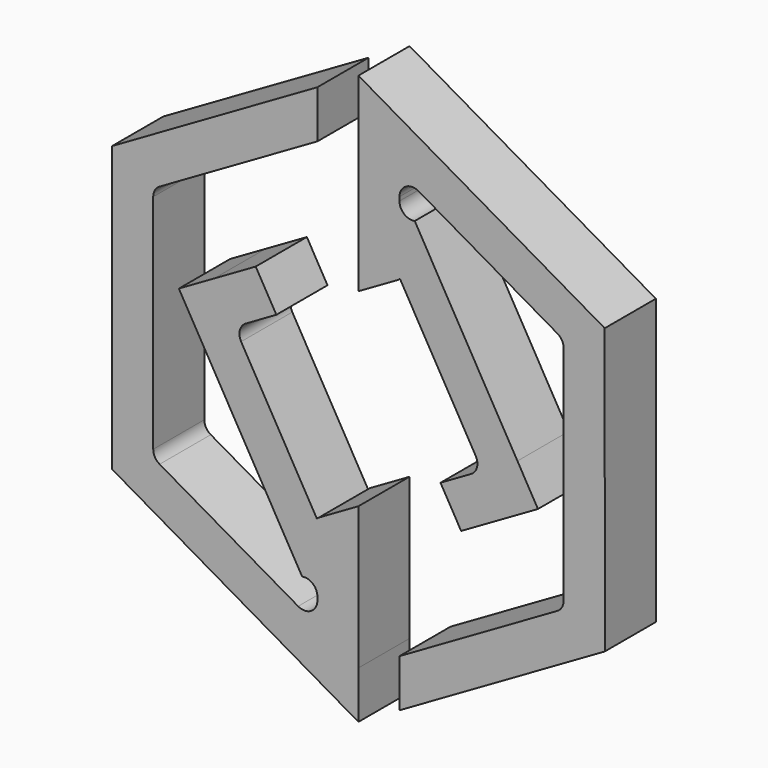
from build123d import *

# Parameters (mm, degrees)
F1_DEPTH      = 25.4
F2_T1_DEPTH   = 25.4
F2_T3_DEPTH   = 31.626178471
F2_2_T1_DEPTH = 25.4
F2_2_T3_DEPTH = 31.595918111


# Not quite as in the source:
# - a fillet or chamfer that OpenCascade refuses, or shapes differently, is made with other operations: its cross-section is extruded or revolved along the edge and cut away or added


with BuildPart() as f1:
    # F0 (on Front) → F1 (new body)
    with BuildSketch(Plane.XZ):
        Polygon((-16.319119, 103.6338542), (-97.871661, 56.5480962), (-97.834323, -56.4841898), (0.000889, -113.0128042), (-0.021209, -94.1582318), (-0.041783, -37.6147838), (-16.454247, -47.0889838), (-16.483203, -47.3297758), (-16.538321, -47.2350338), (-49.133125, 9.2218002), (-32.599503, 18.7691522), (-40.798877, 32.9710542), (-57.263665, 23.4681522), (-71.323581, 15.3475182), (-63.162815, 1.2154662), (-22.370161, -69.4435238), (-16.319119, -65.9487378), (-16.319119, -84.7493098), (-81.509997, -47.1080338), (-81.517109, 47.0517982), (-16.276447, 84.7189822), align=None)
    extrude(amount=F1_DEPTH)

    # F2: fillet of radius 5.08 on 6 edges, made by hand

    # F2_s2 → F2_t1 (join)
    with BuildSketch(Plane.XZ):
        with BuildLine():
            ThreePointArc((-78.9703857887, -48.5744077693), (-80.8295799283, -46.715177806), (-81.5102184992, -44.1754789968))
            Line((-81.5102184992, -44.1754789968), (-81.509997, -47.1080338))
            Line((-81.509997, -47.1080338), (-78.9703857887, -48.5744077693))
        make_face()
        with BuildLine():
            ThreePointArc((-16.319119, -75.9501053756), (-18.8592026389, -80.3495627147), (-23.939286275, -80.3494178464))
            Line((-23.939286275, -80.3494178464), (-16.319119, -84.7493098))
            Line((-16.319119, -84.7493098), (-16.319119, -75.9501053756))
        make_face()
        with BuildLine():
            ThreePointArc((-22.370161, -69.4435238), (-18.1685225659, -70.5094387585), (-16.319119, -74.4298528539))
            Line((-16.319119, -74.4298528539), (-16.319119, -65.9487378))
            Line((-16.319119, -65.9487378), (-22.370161, -69.4435238))
        make_face()
        with BuildLine():
            ThreePointArc((-81.5168874538, 44.1186213446), (-80.8363993057, 46.6588270036), (-78.9769112502, 48.5184003635))
            Line((-78.9769112502, 48.5184003635), (-81.517109, 47.0517982))
            Line((-81.517109, 47.0517982), (-81.5168874538, 44.1186213446))
        make_face()
        with BuildLine():
            ThreePointArc((-46.5933683691, 4.8227365177), (-47.1008880705, 8.6773378396), (-44.7342717126, 11.7619212171))
            Line((-44.7342717126, 11.7619212171), (-49.133125, 9.2218002))
            Line((-49.133125, 9.2218002), (-46.5933683691, 4.8227365177))
        make_face()
    extrude(amount=F2_T1_DEPTH)

    # F2_s4 → F2_t3 (cut)
    with BuildSketch(Plane.XZ.offset(-3.1130892355)):
        with BuildLine():
            ThreePointArc((-15.3757974258, -46.4664418736), (-15.9594734444, -46.8596619247), (-16.483203, -47.3297758))
            Line((-16.483203, -47.3297758), (-16.454247, -47.0889838))
            Line((-16.454247, -47.0889838), (-15.3757974258, -46.4664418736))
        make_face()
    extrude(amount=F2_T3_DEPTH, mode=Mode.SUBTRACT)


with BuildPart() as f1b:
    # F0 (on Front) → F1, piece 2 (new body)
    with BuildSketch(Plane.XZ):
        Polygon((16.316833, -103.6324318), (97.871661, -56.5476898), (97.836101, 56.4845962), (0.000889, 113.0128042), (0.021463, 94.1586382), (0.040767, 37.6151902), (16.451707, 47.0888822), (16.483457, 47.3301822), (16.537305, 47.2326462), (49.133379, -9.2246958), (32.599757, -18.7700158), (40.799131, -32.9709018), (57.261125, -23.4664758), (71.323835, -15.3499058), (63.164339, -1.2178538), (22.370669, 69.4408822), (16.316833, 65.9488902), (16.316833, 84.7479382), (81.507711, 47.1056462), (81.518633, -47.0516458), (16.278225, -84.7203538), align=None)
    extrude(amount=F1_DEPTH)

    # F2#2: fillet of radius 5.08 on 6 edges, made by hand

    # F2_2_s2 → F2_2_t1 (join)
    with BuildSketch(Plane.XZ):
        with BuildLine():
            ThreePointArc((46.5932982219, -4.8252024991), (47.1007988179, -8.6800552118), (44.7338290233, -11.7646784114))
            Line((44.7338290233, -11.7646784114), (49.133379, -9.2246958))
            Line((49.133379, -9.2246958), (46.5932982219, -4.8252024991))
        make_face()
        with BuildLine():
            ThreePointArc((16.316833, 75.9486150149), (18.8569423497, 80.3480871974), (23.9370516947, 80.3478977955))
            Line((23.9370516947, 80.3478977955), (16.316833, 84.7479382))
            Line((16.316833, 84.7479382), (16.316833, 75.9486150149))
        make_face()
        with BuildLine():
            ThreePointArc((22.370669, 69.4408822), (18.1673351195, 70.505347241), (16.316833, 74.4266663354))
            Line((16.316833, 74.4266663354), (16.316833, 65.9488902))
            Line((16.316833, 65.9488902), (22.370669, 69.4408822))
        make_face()
        with BuildLine():
            ThreePointArc((78.968269877, 48.5719615374), (80.8273760471, 46.7128245665), (81.5080511482, 44.1732680235))
            Line((81.5080511482, 44.1732680235), (81.507711, 47.1056462))
            Line((81.507711, 47.1056462), (78.968269877, 48.5719615374))
        make_face()
        with BuildLine():
            ThreePointArc((78.9784010584, -48.5183327536), (80.8378803981, -46.6586769125), (81.5182927508, -44.1183969491))
            Line((81.5182927508, -44.1183969491), (81.518633, -47.0516458))
            Line((81.518633, -47.0516458), (78.9784010584, -48.5183327536))
        make_face()
    extrude(amount=F2_2_T1_DEPTH)

    # F2_2_s4 → F2_2_t3 (cut)
    with BuildSketch(Plane.XZ.offset(-3.0979590555)):
        with BuildLine():
            ThreePointArc((15.3785094128, 46.4693477068), (15.9607949827, 46.861499235), (16.483457, 47.3301822))
            Line((16.483457, 47.3301822), (16.451707, 47.0888822))
            Line((16.451707, 47.0888822), (15.3785094128, 46.4693477068))
        make_face()
    extrude(amount=F2_2_T3_DEPTH, mode=Mode.SUBTRACT)


solid = Compound([f1.part, f1b.part])
